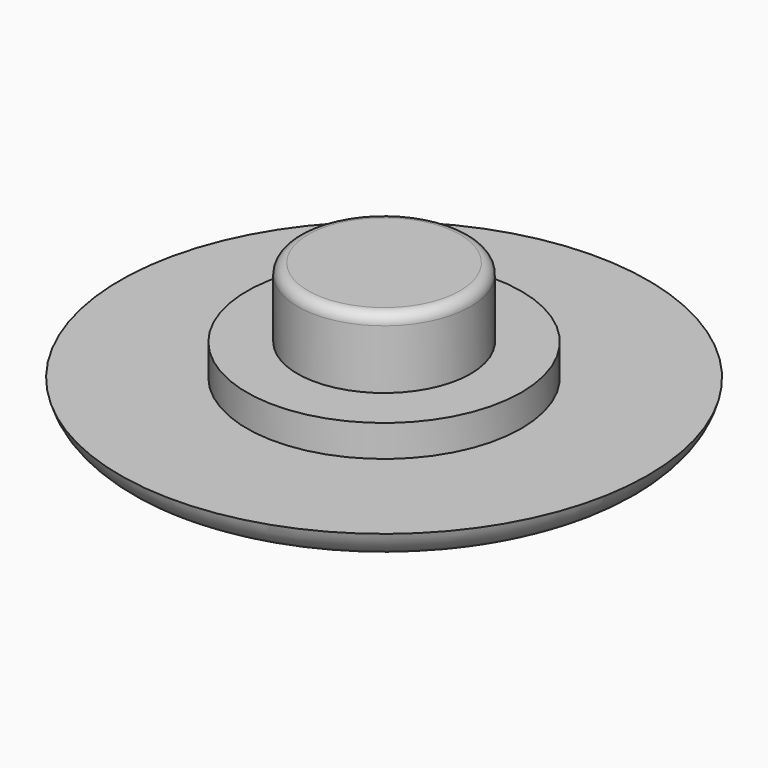
from build123d import *

# Parameters (mm, degrees)
F0_R     = 4.1
F1_DEPTH = 6.3
F0_R_2   = 6.5
F2_DEPTH = 3
F0_R_3   = 12.5
F3_DEPTH = 1.5
F4_R     = 0.5


# Not quite as in the source:
# - a fillet or chamfer that OpenCascade refuses, or shapes differently, is made with other operations: its cross-section is extruded or revolved along the edge and cut away or added
# - a feature names something its author has since deleted; it is built from what else it names


with BuildPart() as f1:
    # F0 (on Top) → F1 (new body)
    with BuildSketch(Plane.XY):
        Circle(F0_R)
    extrude(amount=F1_DEPTH)

    # F0 (on Top) → F2 (join)
    with BuildSketch(Plane.XY):
        Circle(F0_R_2)
        Circle(F0_R, mode=Mode.SUBTRACT)
    extrude(amount=F2_DEPTH)

    # F0 (on Top) → F3 (join)
    with BuildSketch(Plane.XY):
        Circle(F0_R_3)
        Circle(F0_R_2, mode=Mode.SUBTRACT)
    extrude(amount=F3_DEPTH)

    # F4
    f4_edges = [f1.edges().sort_by_distance(p)[0] for p in [
        (-4.1, 0, 6.3),
    ]]
    fillet(f4_edges, radius=F4_R)

    # F5: fillet of radius 2 on 1 edges, made by hand

    # F5_s1 → F5_t2 (revolve, cut)
    with BuildSketch(Plane.XZ):
        with BuildLine():
            ThreePointArc((12.5, 1.5), (11.7882531983, 0.4188611699), (10.5635083269, 0))
            Line((10.5635083269, 0), (12.5, 0))
            Line((12.5, 0), (12.5, 1.5))
        make_face()
    revolve(axis=Axis((0, 0, 0), (0, 0, 1)), mode=Mode.SUBTRACT)


solid = f1.part
